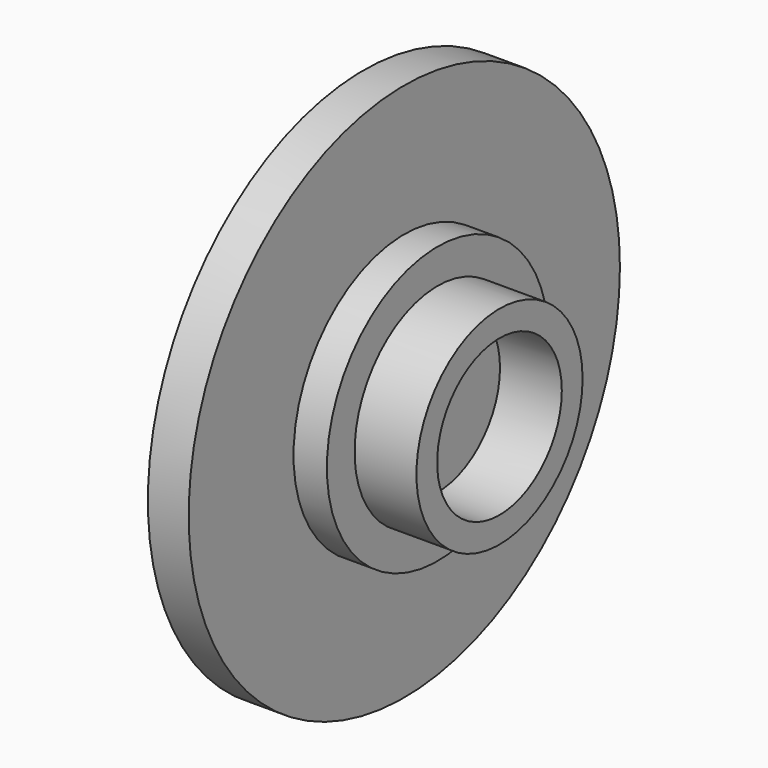
from build123d import *

# Parameters (mm, degrees)
F0_R      = 10.9
F1_DEPTH  = 1.65
F2_R      = 4.2
F3_DEPTH  = 5.5
F5_R      = 3.15
F6_DEPTH  = 3.37
F7_R      = 3.18
F8_DEPTH  = 1.65
F9_R      = 5.6
F10_DEPTH = 3


# Not quite as in the source:
# - a feature names something its author has since deleted; it is built from what else it names


with BuildPart() as f1:
    # F0 (on Right) → F1 (new body)
    with BuildSketch(Plane.YZ):
        Circle(F0_R)
    extrude(amount=F1_DEPTH)

    # F2 (on Right) → F3 (join)
    with BuildSketch(Plane.YZ):
        Circle(F2_R)
    extrude(amount=F3_DEPTH)

    # F5 (on offset) → F6 (cut)
    with BuildSketch(Plane.YZ.offset(5.5)):
        Circle(F5_R)
    extrude(amount=-F6_DEPTH, mode=Mode.SUBTRACT)

    # F7 (on Right) → F8 (join)
    with BuildSketch(Plane.YZ):
        Circle(F7_R)
    extrude(amount=F8_DEPTH)

    # F9 (on Right) → F10 (join)
    with BuildSketch(Plane.YZ):
        Circle(F9_R)
    extrude(amount=F10_DEPTH)


solid = f1.part
